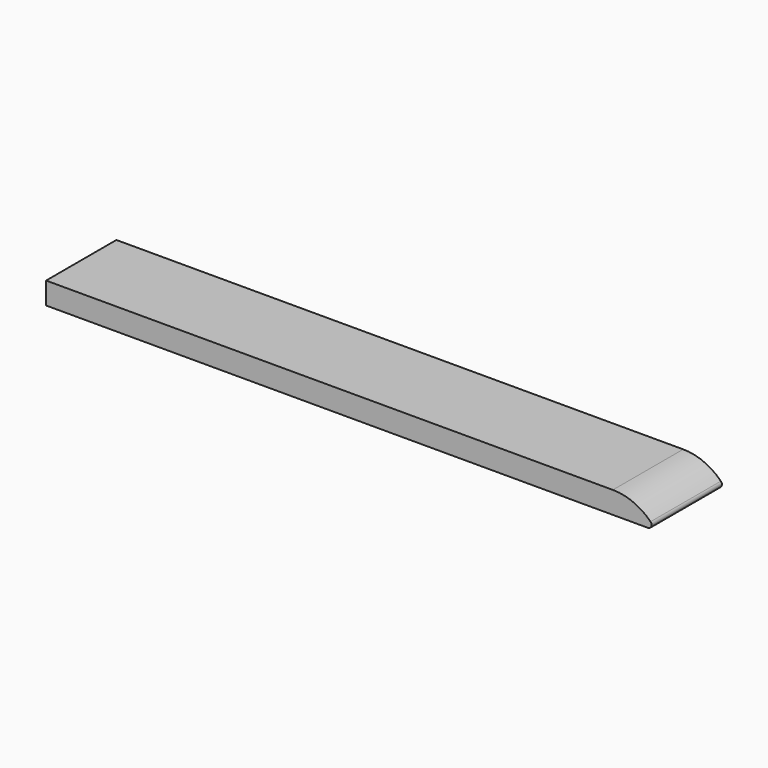
from build123d import *

# Parameters (mm, degrees)
F0_W        = 704.85
F0_H        = 101.6
F1_DEPTH    = 25.4
F2_T1_DEPTH = 350.0928592435
F3_R        = 4.2426380505


# Not quite as in the source:
# - a fillet or chamfer that OpenCascade refuses, or shapes differently, is made with other operations: its cross-section is extruded or revolved along the edge and cut away or added


with BuildPart() as f1:
    # F0 (on Top) → F1 (new body)
    with BuildSketch(Plane.XY):
        with Locations((25.5663767457, 11.9668386396)):
            Rectangle(F0_W, F0_H)
    extrude(amount=F1_DEPTH)

    # F2: fillet of radius 61.3210244843 on 1 edges, made by hand

    # F2_s2 → F2_t1 (cut)
    with BuildSketch(Plane.XZ.offset(-187.0132682614)):
        with BuildLine():
            ThreePointArc((377.9913767457, 0), (356.1993813791, 18.6820068679), (328.292804897, 25.4))
            Line((328.292804897, 25.4), (377.9913767457, 25.4))
            Line((377.9913767457, 25.4), (377.9913767457, 0))
        make_face()
    extrude(amount=F2_T1_DEPTH, mode=Mode.SUBTRACT)

    # F3
    f3_edges = [f1.edges().sort_by_distance(p)[0] for p in [
        (377.991377, 11.966839, 0),
    ]]
    fillet(f3_edges, radius=F3_R)


solid = f1.part
